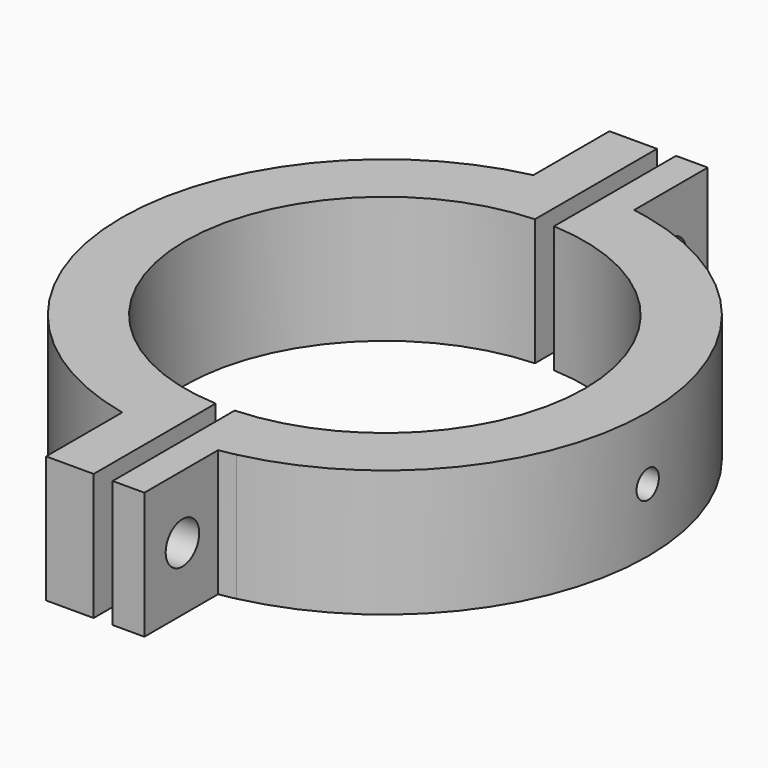
from build123d import *

# Parameters (mm, degrees)
F0_R                 = 31.5
F1_DEPTH             = 10
F1_DEPTH_BACK        = 10
F3_DEPTH             = 20
F6_D                 = 6.6
F6_CBORE_D           = 11.25
F6_CBORE_DEPTH       = 6
F6_ON_F5_D           = 6.6
F6_ON_F5_CBORE_D     = 11.25
F6_ON_F5_CBORE_DEPTH = 6
F11_D                = 4.4
F11_DEPTH            = 14.25
F11_START            = 2.0000001
F11_CBORE_D          = 8.25
F11_CBORE_DEPTH      = 6
F11_TIP              = 1.3218933619


# Not quite as in the source:
# - a feature names something its author has since deleted; it is built from what else it names


with BuildPart() as f1:
    # F0 (on Top) → F1 (new body, two sides)
    with BuildSketch(Plane.XY) as f1_sk:
        with BuildLine():
            ThreePointArc((9, -40.5123437979), (32.3708974235, -25.9687311973), (41.5, 0))
            ThreePointArc((41.5, 0), (32.3708974235, 25.9687311973), (9, 40.5123437979))
            Line((9, 40.5123437979), (-9, 40.5123437979))
            ThreePointArc((-9, 40.5123437979), (-41.5, 0), (-9, -40.5123437979))
            Line((-9, -40.5123437979), (9, -40.5123437979))
        make_face()
        Circle(F0_R, mode=Mode.SUBTRACT)
        with BuildLine():
            ThreePointArc((-9, 40.5123437979), (0, 41.5), (9, 40.5123437979))
            Line((9, 40.5123437979), (9, 55.5123437979))
            Line((9, 55.5123437979), (-9, 55.5123437979))
            Line((-9, 55.5123437979), (-9, 40.5123437979))
        make_face()
        with BuildLine():
            Line((9, -55.5123437979), (9, -40.5123437979))
            ThreePointArc((9, -40.5123437979), (0, -41.5), (-9, -40.5123437979))
            Line((-9, -40.5123437979), (-9, -55.5123437979))
            Line((-9, -55.5123437979), (9, -55.5123437979))
        make_face()
        with BuildLine():
            ThreePointArc((-9, -40.5123437979), (0, -41.5), (9, -40.5123437979))
            Line((9, -40.5123437979), (-9, -40.5123437979))
        make_face()
        with BuildLine():
            Line((-9, 40.5123437979), (9, 40.5123437979))
            ThreePointArc((9, 40.5123437979), (0, 41.5), (-9, 40.5123437979))
        make_face()
    extrude(amount=F1_DEPTH)
    extrude(f1_sk.sketch, amount=-F1_DEPTH_BACK)

    # F2 (on face) → F3 (cut, through all)
    with BuildSketch(Plane.XY.offset(10)):
        with BuildLine():
            ThreePointArc((1.5, -41.4728827067), (0, -41.5), (-1.5, -41.4728827067))
            Line((-1.5, -41.4728827067), (-1.5, -55.5123437979))
            Line((-1.5, -55.5123437979), (1.5, -55.5123437979))
            Line((1.5, -55.5123437979), (1.5, -41.4728827067))
        make_face()
        with BuildLine():
            ThreePointArc((1.5, -31.4642654451), (0, -31.5), (-1.5, -31.4642654451))
            Line((-1.5, -31.4642654451), (-1.5, -41.4728827067))
            ThreePointArc((-1.5, -41.4728827067), (0, -41.5), (1.5, -41.4728827067))
            Line((1.5, -41.4728827067), (1.5, -31.4642654451))
        make_face()
        with BuildLine():
            Line((9, -55.5123437979), (9, -40.5123437979))
            ThreePointArc((9, -40.5123437979), (7.7536452961, -40.7692406677), (6.5, -40.9878030638))
            Line((6.5, -40.9878030638), (6.5, -55.5123437979))
            Line((6.5, -55.5123437979), (9, -55.5123437979))
        make_face()
        with BuildLine():
            Line((1.5, 55.5123437979), (-1.5, 55.5123437979))
            Line((-1.5, 55.5123437979), (-1.5, 41.4728827067))
            ThreePointArc((-1.5, 41.4728827067), (0, 41.5), (1.5, 41.4728827067))
            Line((1.5, 41.4728827067), (1.5, 55.5123437979))
        make_face()
        with BuildLine():
            ThreePointArc((1.5, 41.4728827067), (0, 41.5), (-1.5, 41.4728827067))
            Line((-1.5, 41.4728827067), (-1.5, 31.4642654451))
            ThreePointArc((-1.5, 31.4642654451), (0, 31.5), (1.5, 31.4642654451))
            Line((1.5, 31.4642654451), (1.5, 41.4728827067))
        make_face()
        with BuildLine():
            Line((9, 55.5123437979), (6.5, 55.5123437979))
            Line((6.5, 55.5123437979), (6.5, 40.9878030638))
            ThreePointArc((6.5, 40.9878030638), (7.7536452961, 40.7692406677), (9, 40.5123437979))
            Line((9, 40.5123437979), (9, 55.5123437979))
        make_face()
    extrude(amount=-F3_DEPTH, mode=Mode.SUBTRACT)

    # F6 (through all)
    with Locations(Plane(origin=(-9, 0, 0), x_dir=(0, -1, 0), z_dir=(-1, 0, 0))):
        with Locations((-48.0123437979, 0)):
            CounterBoreHole(F6_D / 2, F6_CBORE_D / 2, F6_CBORE_DEPTH)

    # F6 on F5 (through all)
    with Locations(Plane(origin=(-9, 0, 0), x_dir=(0, -1, 0), z_dir=(-1, 0, 0))):
        with Locations((48.0123437979, 0)):
            CounterBoreHole(F6_ON_F5_D / 2, F6_ON_F5_CBORE_D / 2, F6_ON_F5_CBORE_DEPTH)

    # F11
    # its depths count from where the whole tool has entered the part; down to there all is cleared
    with Locations(Plane(origin=(29.5, 0, 0), x_dir=(0, -1, 0), z_dir=(-1, 0, 0)).offset(-F11_START)):
        with Locations((0, 0)):
            CounterBoreHole(F11_D / 2, F11_CBORE_D / 2, F11_CBORE_DEPTH, depth=F11_DEPTH)
            with Locations((0, 0, -(F11_DEPTH + F11_TIP / 2))):  # 118° drill point
                Cone(0, F11_D / 2, F11_TIP, mode=Mode.SUBTRACT)


solid = f1.part
